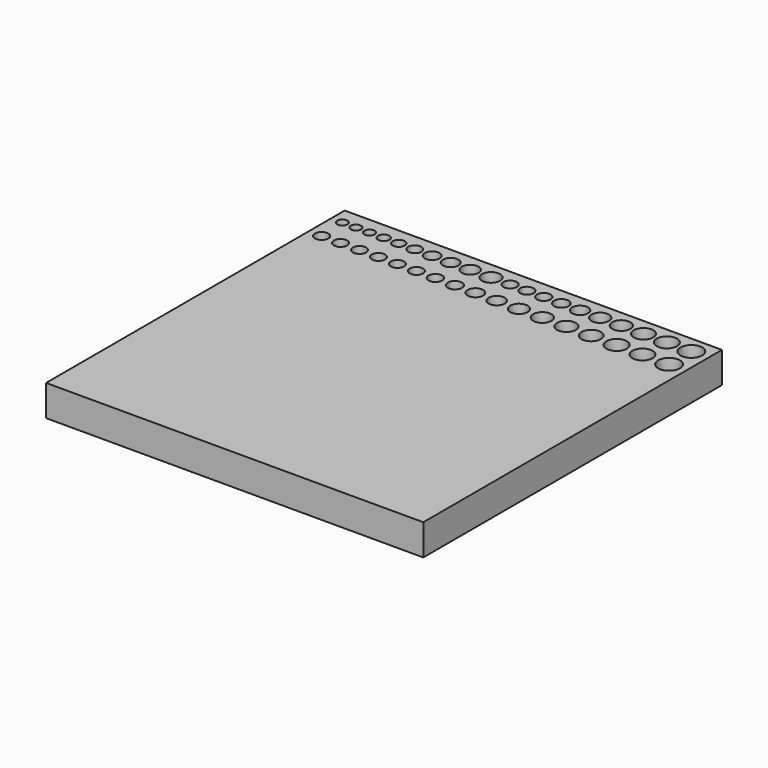
from build123d import *

# Parameters (mm, degrees)
F0_W     = 617.5375
F0_H     = 611.12411
F1_DEPTH = 50.8
F2_DEPTH = 25.4


# Not quite as in the source:
# - the dataset's text gives a spline's control points without its knots; the knots are read off the source's solid


with BuildPart() as f1:
    # F0 (on Top) → F1 (new body)
    with BuildSketch(Plane.XY):
        Rectangle(F0_W, F0_H)
        with BuildLine():
            add(Edge.make_bspline(
                [(-298.769016, 232.10194), (-298.769016, 238.169097), (-293.850797, 243.087316), (-287.783984, 243.087316), (-281.716482, 243.087316), (-276.798953, 238.169097), (-276.798953, 232.10194), (-276.798953, 226.035126), (-281.716482, 221.117253), (-287.783984, 221.117253), (-293.850797, 221.117253), (-298.769016, 226.035126), (-298.769016, 232.10194)],
                knots=[0, 0, 0, 0, 1, 1, 1, 2, 2, 2, 3, 3, 3, 4, 4, 4, 4], degree=3))
        make_face(mode=Mode.SUBTRACT)
        with BuildLine():
            add(Edge.make_bspline(
                [(-267.73973, 232.10194), (-267.73973, 238.158073), (-262.831158, 243.067334), (-256.77468, 243.067334), (-250.718891, 243.067334), (-245.80963, 238.158073), (-245.80963, 232.10194), (-245.80963, 226.046151), (-250.718891, 221.137234), (-256.77468, 221.137234), (-262.831158, 221.137234), (-267.73973, 226.046151), (-267.73973, 232.10194)],
                knots=[0, 0, 0, 0, 1, 1, 1, 2, 2, 2, 3, 3, 3, 4, 4, 4, 4], degree=3))
        make_face(mode=Mode.SUBTRACT)
        with BuildLine():
            add(Edge.make_bspline(
                [(-298.769016, 277.737052), (-298.769016, 282.365194), (-295.017651, 286.117247), (-290.389165, 286.117247), (-285.761024, 286.117247), (-282.008971, 282.365194), (-282.008971, 277.737052), (-282.008971, 273.108911), (-285.761024, 269.356858), (-290.389165, 269.356858), (-295.017651, 269.356858), (-298.769016, 273.108911), (-298.769016, 277.737052)],
                knots=[0, 0, 0, 0, 1, 1, 1, 2, 2, 2, 3, 3, 3, 4, 4, 4, 4], degree=3))
        make_face(mode=Mode.SUBTRACT)
        with BuildLine():
            add(Edge.make_bspline(
                [(-276.498885, 277.737052), (-276.498885, 282.362438), (-272.749588, 286.11208), (-268.123858, 286.11208), (-263.498473, 286.11208), (-259.748831, 282.362438), (-259.748831, 277.737052), (-259.748831, 273.111667), (-263.498473, 269.362025), (-268.123858, 269.362025), (-272.749588, 269.362025), (-276.498885, 273.111667), (-276.498885, 277.737052)],
                knots=[0, 0, 0, 0, 1, 1, 1, 2, 2, 2, 3, 3, 3, 4, 4, 4, 4], degree=3))
        make_face(mode=Mode.SUBTRACT)
        with BuildLine():
            add(Edge.make_bspline(
                [(-254.238745, 277.737052), (-254.238745, 282.398611), (-250.460509, 286.177192), (-245.79895, 286.177192), (-241.137736, 286.177192), (-237.359155, 282.398611), (-237.359155, 277.737052), (-237.359155, 273.075838), (-241.137736, 269.296913), (-245.79895, 269.296913), (-250.460509, 269.296913), (-254.238745, 273.075838), (-254.238745, 277.737052)],
                knots=[0, 0, 0, 0, 1, 1, 1, 2, 2, 2, 3, 3, 3, 4, 4, 4, 4], degree=3))
        make_face(mode=Mode.SUBTRACT)
        with BuildLine():
            add(Edge.make_bspline(
                [(-236.750407, 232.10194), (-236.750407, 238.163585), (-231.837012, 243.077325), (-225.775711, 243.077325), (-219.71441, 243.077325), (-214.800325, 238.163585), (-214.800325, 232.10194), (-214.800325, 226.040639), (-219.71441, 221.127243), (-225.775711, 221.127243), (-231.837012, 221.127243), (-236.750407, 226.040639), (-236.750407, 232.10194)],
                knots=[0, 0, 0, 0, 1, 1, 1, 2, 2, 2, 3, 3, 3, 4, 4, 4, 4], degree=3))
        make_face(mode=Mode.SUBTRACT)
        with BuildLine():
            add(Edge.make_bspline(
                [(-205.741102, 232.102284), (-205.741102, 238.17771), (-200.816683, 243.102474), (-194.740912, 243.102474), (-188.665831, 243.102474), (-183.741412, 238.17771), (-183.741412, 232.102284), (-183.741412, 226.027203), (-188.665831, 221.102439), (-194.740912, 221.102439), (-200.816683, 221.102439), (-205.741102, 226.027203), (-205.741102, 232.102284)],
                knots=[0, 0, 0, 0, 1, 1, 1, 2, 2, 2, 3, 3, 3, 4, 4, 4, 4], degree=3))
        make_face(mode=Mode.SUBTRACT)
        with BuildLine():
            add(Edge.make_bspline(
                [(-174.682188, 232.10194), (-174.682188, 238.17771), (-169.75708, 243.102474), (-163.681999, 243.102474), (-157.606917, 243.102474), (-152.681809, 238.17771), (-152.681809, 232.10194), (-152.681809, 226.026858), (-157.606917, 221.102094), (-163.681999, 221.102094), (-169.75708, 221.102094), (-174.682188, 226.026858), (-174.682188, 232.10194)],
                knots=[0, 0, 0, 0, 1, 1, 1, 2, 2, 2, 3, 3, 3, 4, 4, 4, 4], degree=3))
        make_face(mode=Mode.SUBTRACT)
        with BuildLine():
            add(Edge.make_bspline(
                [(-231.849414, 277.73688), (-231.849414, 282.848368), (-227.705998, 286.992129), (-222.594509, 286.992129), (-217.482677, 286.992129), (-213.33926, 282.848368), (-213.33926, 277.73688), (-213.33926, 272.625392), (-217.482677, 268.481976), (-222.594509, 268.481976), (-227.705998, 268.481976), (-231.849414, 272.625392), (-231.849414, 277.73688)],
                knots=[0, 0, 0, 0, 1, 1, 1, 2, 2, 2, 3, 3, 3, 4, 4, 4, 4], degree=3))
        make_face(mode=Mode.SUBTRACT)
        with BuildLine():
            add(Edge.make_bspline(
                [(-198.029256179, 287.5369713483), (-192.616666179, 287.5369712893), (-188.2293372268, 283.1496422416), (-188.2293372857, 277.7370522416), (-188.2293373447, 272.3244632416), (-192.6166663924, 267.9371332893), (-198.0292563924, 267.9371333483), (-203.4418453924, 267.9371334072), (-207.8291743447, 272.324463455), (-207.8291742857, 277.737052455), (-207.8291742268, 283.149642455), (-203.441845179, 287.5369714072), (-198.029256179, 287.5369713483)],
                knots=[0, 0, 0, 0, 1, 1, 1, 2, 2, 2, 3, 3, 3, 4, 4, 4, 4], degree=3))
        make_face(mode=Mode.SUBTRACT)
        with BuildLine():
            add(Edge.make_bspline(
                [(-182.719596, 277.737052), (-182.719596, 283.759424), (-177.837207, 288.641813), (-171.814491, 288.641813), (-165.792464, 288.641813), (-160.90973, 283.759424), (-160.90973, 277.737052), (-160.90973, 271.714681), (-165.792464, 266.832292), (-171.814491, 266.832292), (-177.837207, 266.832292), (-182.719596, 271.714681), (-182.719596, 277.737052)],
                knots=[0, 0, 0, 0, 1, 1, 1, 2, 2, 2, 3, 3, 3, 4, 4, 4, 4], degree=3))
        make_face(mode=Mode.SUBTRACT)
        with BuildLine():
            add(Edge.make_bspline(
                [(-143.622586, 232.10194), (-143.622586, 238.144293), (-138.725038, 243.042529), (-132.68234, 243.042529), (-126.640332, 243.042529), (-121.742784, 238.144293), (-121.742784, 232.10194), (-121.742784, 226.059931), (-126.640332, 221.162039), (-132.68234, 221.162039), (-138.725038, 221.162039), (-143.622586, 226.059931), (-143.622586, 232.10194)],
                knots=[0, 0, 0, 0, 1, 1, 1, 2, 2, 2, 3, 3, 3, 4, 4, 4, 4], degree=3))
        make_face(mode=Mode.SUBTRACT)
        with BuildLine():
            add(Edge.make_bspline(
                [(-112.683561, 232.102284), (-112.683561, 238.260737), (-107.692307, 243.25268), (-101.533854, 243.25268), (-95.375401, 243.25268), (-90.383458, 238.260737), (-90.383458, 232.102284), (-90.383458, 225.94452), (-95.375401, 220.952233), (-101.533854, 220.952233), (-107.692307, 220.952233), (-112.683561, 225.94452), (-112.683561, 232.102284)],
                knots=[0, 0, 0, 0, 1, 1, 1, 2, 2, 2, 3, 3, 3, 4, 4, 4, 4], degree=3))
        make_face(mode=Mode.SUBTRACT)
        with BuildLine():
            add(Edge.make_bspline(
                [(-155.399645, 277.737052), (-155.399645, 284.402968), (-149.995668, 289.806945), (-143.329408, 289.806945), (-136.663837, 289.806945), (-131.259516, 284.402968), (-131.259516, 277.737052), (-131.259516, 271.071137), (-136.663837, 265.66716), (-143.329408, 265.66716), (-149.995668, 265.66716), (-155.399645, 271.071137), (-155.399645, 277.737052)],
                knots=[0, 0, 0, 0, 1, 1, 1, 2, 2, 2, 3, 3, 3, 4, 4, 4, 4], degree=3))
        make_face(mode=Mode.SUBTRACT)
        with BuildLine():
            add(Edge.make_bspline(
                [(-112.9898302501, 290.4969974494), (-105.9425422501, 290.4969974298), (-100.2298852661, 284.7843394139), (-100.2298852857, 277.7370524139), (-100.2298853054, 270.6897654139), (-105.9425423213, 264.9771074298), (-112.9898303213, 264.9771074494), (-120.0371173213, 264.9771074691), (-125.7497743054, 270.689765485), (-125.7497742857, 277.737052485), (-125.7497742661, 284.784339485), (-120.0371172501, 290.4969974691), (-112.9898302501, 290.4969974494)],
                knots=[0, 0, 0, 0, 1, 1, 1, 2, 2, 2, 3, 3, 3, 4, 4, 4, 4], degree=3))
        make_face(mode=Mode.SUBTRACT)
        with BuildLine():
            add(Edge.make_bspline(
                [(-94.7198, 277.737052), (-94.7198, 285.305927), (-88.584085, 291.441987), (-81.014865, 291.441987), (-73.446335, 291.441987), (-67.309931, 285.305927), (-67.309931, 277.737052), (-67.309931, 270.168178), (-73.446335, 264.032118), (-81.014865, 264.032118), (-88.584085, 264.032118), (-94.7198, 270.168178), (-94.7198, 277.737052)],
                knots=[0, 0, 0, 0, 1, 1, 1, 2, 2, 2, 3, 3, 3, 4, 4, 4, 4], degree=3))
        make_face(mode=Mode.SUBTRACT)
        with BuildLine():
            add(Edge.make_bspline(
                [(-81.324235, 232.102284), (-81.324235, 238.583887), (-76.071153, 243.837657), (-69.589551, 243.837657), (-63.107948, 243.837657), (-57.854177, 238.583887), (-57.854177, 232.102284), (-57.854177, 225.621371), (-63.107948, 220.367255), (-69.589551, 220.367255), (-76.071153, 220.367255), (-81.324235, 225.621371), (-81.324235, 232.102284)],
                knots=[0, 0, 0, 0, 1, 1, 1, 2, 2, 2, 3, 3, 3, 4, 4, 4, 4], degree=3))
        make_face(mode=Mode.SUBTRACT)
        with BuildLine():
            add(Edge.make_bspline(
                [(-48.794954, 232.10194), (-48.794954, 239.11891), (-43.106413, 244.807107), (-36.089442, 244.807107), (-29.073161, 244.807107), (-23.384619, 239.11891), (-23.384619, 232.10194), (-23.384619, 225.085658), (-29.073161, 219.397461), (-36.089442, 219.397461), (-43.106413, 219.397461), (-48.794954, 225.085658), (-48.794954, 232.10194)],
                knots=[0, 0, 0, 0, 1, 1, 1, 2, 2, 2, 3, 3, 3, 4, 4, 4, 4], degree=3))
        make_face(mode=Mode.SUBTRACT)
        with BuildLine():
            add(Edge.make_bspline(
                [(-14.325396, 232.10194), (-14.325396, 239.353866), (-8.447374, 245.232232), (-1.195448, 245.232232), (6.055789, 245.232232), (11.9345, 239.353866), (11.9345, 232.10194), (11.9345, 224.850703), (6.055789, 218.971992), (-1.195448, 218.971992), (-8.447374, 218.971992), (-14.325396, 224.850703), (-14.325396, 232.10194)],
                knots=[0, 0, 0, 0, 1, 1, 1, 2, 2, 2, 3, 3, 3, 4, 4, 4, 4], degree=3))
        make_face(mode=Mode.SUBTRACT)
        with BuildLine():
            add(Edge.make_bspline(
                [(-61.80019, 277.737052), (-61.80019, 285.919154), (-55.167347, 292.551997), (-46.985246, 292.551997), (-38.803144, 292.551997), (-32.169957, 285.919154), (-32.169957, 277.737052), (-32.169957, 269.554951), (-38.803144, 262.922108), (-46.985246, 262.922108), (-55.167347, 262.922108), (-61.80019, 269.554951), (-61.80019, 277.737052)],
                knots=[0, 0, 0, 0, 1, 1, 1, 2, 2, 2, 3, 3, 3, 4, 4, 4, 4], degree=3))
        make_face(mode=Mode.SUBTRACT)
        with BuildLine():
            add(Edge.make_bspline(
                [(-26.66056, 277.737052), (-26.66056, 283.80111), (-21.745098, 288.716916), (-15.681041, 288.716916), (-9.616984, 288.716916), (-4.700833, 283.80111), (-4.700833, 277.737052), (-4.700833, 271.672995), (-9.616984, 266.757189), (-15.681041, 266.757189), (-21.745098, 266.757189), (-26.66056, 271.672995), (-26.66056, 277.737052)],
                knots=[0, 0, 0, 0, 1, 1, 1, 2, 2, 2, 3, 3, 3, 4, 4, 4, 4], degree=3))
        make_face(mode=Mode.SUBTRACT)
        with BuildLine():
            add(Edge.make_bspline(
                [(20.993723, 232.101595), (20.993723, 239.974672), (27.375762, 246.357056), (35.248495, 246.357056), (43.120882, 246.357056), (49.503266, 239.974672), (49.503266, 232.101595), (49.503266, 224.229207), (43.120882, 217.846824), (35.248495, 217.846824), (27.375762, 217.846824), (20.993723, 224.229207), (20.993723, 232.101595)],
                knots=[0, 0, 0, 0, 1, 1, 1, 2, 2, 2, 3, 3, 3, 4, 4, 4, 4], degree=3))
        make_face(mode=Mode.SUBTRACT)
        with BuildLine():
            add(Edge.make_bspline(
                [(58.562489, 232.101595), (58.562489, 240.350187), (65.249075, 247.037118), (73.497667, 247.037118), (81.74557, 247.037118), (88.432501, 240.350187), (88.432501, 232.101595), (88.432501, 223.853692), (81.74557, 217.166762), (73.497667, 217.166762), (65.249075, 217.166762), (58.562489, 223.853692), (58.562489, 232.101595)],
                knots=[0, 0, 0, 0, 1, 1, 1, 2, 2, 2, 3, 3, 3, 4, 4, 4, 4], degree=3))
        make_face(mode=Mode.SUBTRACT)
        with BuildLine():
            add(Edge.make_bspline(
                [(0.808908, 277.737052), (0.808908, 283.812134), (5.733328, 288.736898), (11.809098, 288.736898), (17.88418, 288.736898), (22.808599, 283.812134), (22.808599, 277.737052), (22.808599, 271.661971), (17.88418, 266.737207), (11.809098, 266.737207), (5.733328, 266.737207), (0.808908, 271.661971), (0.808908, 277.737052)],
                knots=[0, 0, 0, 0, 1, 1, 1, 2, 2, 2, 3, 3, 3, 4, 4, 4, 4], degree=3))
        make_face(mode=Mode.SUBTRACT)
        with BuildLine():
            add(Edge.make_bspline(
                [(28.318685, 277.737052), (28.318685, 283.87828), (33.296848, 288.857132), (39.438764, 288.857132), (45.579991, 288.857132), (50.558843, 283.87828), (50.558843, 277.737052), (50.558843, 271.595825), (45.579991, 266.616973), (39.438764, 266.616973), (33.296848, 266.616973), (28.318685, 271.595825), (28.318685, 277.737052)],
                knots=[0, 0, 0, 0, 1, 1, 1, 2, 2, 2, 3, 3, 3, 4, 4, 4, 4], degree=3))
        make_face(mode=Mode.SUBTRACT)
        with BuildLine():
            add(Edge.make_bspline(
                [(56.068929, 277.737052), (56.068929, 284.380919), (61.454991, 289.766981), (68.099203, 289.766981), (74.742725, 289.766981), (80.128787, 284.380919), (80.128787, 277.737052), (80.128787, 271.093186), (74.742725, 265.707124), (68.099203, 265.707124), (61.454991, 265.707124), (56.068929, 271.093186), (56.068929, 277.737052)],
                knots=[0, 0, 0, 0, 1, 1, 1, 2, 2, 2, 3, 3, 3, 4, 4, 4, 4], degree=3))
        make_face(mode=Mode.SUBTRACT)
        with BuildLine():
            add(Edge.make_bspline(
                [(97.491724, 232.10194), (97.491724, 240.673682), (104.440481, 247.622095), (113.011879, 247.622095), (121.583276, 247.622095), (128.532034, 240.673682), (128.532034, 232.10194), (128.532034, 223.530542), (121.583276, 216.582129), (113.011879, 216.582129), (104.440481, 216.582129), (97.491724, 223.530542), (97.491724, 232.10194)],
                knots=[0, 0, 0, 0, 1, 1, 1, 2, 2, 2, 3, 3, 3, 4, 4, 4, 4], degree=3))
        make_face(mode=Mode.SUBTRACT)
        with BuildLine():
            add(Edge.make_bspline(
                [(137.591257, 232.101595), (137.591257, 240.883488), (144.710202, 248.002089), (153.491062, 248.002089), (162.27261, 248.002089), (169.390866, 240.883488), (169.390866, 232.101595), (169.390866, 223.320736), (162.27261, 216.20179), (153.491062, 216.20179), (144.710202, 216.20179), (137.591257, 223.320736), (137.591257, 232.101595)],
                knots=[0, 0, 0, 0, 1, 1, 1, 2, 2, 2, 3, 3, 3, 4, 4, 4, 4], degree=3))
        make_face(mode=Mode.SUBTRACT)
        with BuildLine():
            add(Edge.make_bspline(
                [(85.638873, 277.737052), (85.638873, 284.994146), (91.521718, 290.876991), (98.778467, 290.876991), (106.035216, 290.876991), (111.91875, 284.994146), (111.91875, 277.737052), (111.91875, 270.479959), (106.035216, 264.597114), (98.778467, 264.597114), (91.521718, 264.597114), (85.638873, 270.479959), (85.638873, 277.737052)],
                knots=[0, 0, 0, 0, 1, 1, 1, 2, 2, 2, 3, 3, 3, 4, 4, 4, 4], degree=3))
        make_face(mode=Mode.SUBTRACT)
        with BuildLine():
            add(Edge.make_bspline(
                [(117.428836, 277.737052), (117.428836, 285.615297), (123.815354, 292.002159), (131.694287, 292.002159), (139.572531, 292.002159), (145.959049, 285.615297), (145.959049, 277.737052), (145.959049, 269.858808), (139.572531, 263.471946), (131.694287, 263.471946), (123.815354, 263.471946), (117.428836, 269.858808), (117.428836, 277.737052)],
                knots=[0, 0, 0, 0, 1, 1, 1, 2, 2, 2, 3, 3, 3, 4, 4, 4, 4], degree=3))
        make_face(mode=Mode.SUBTRACT)
        with BuildLine():
            add(Edge.make_bspline(
                [(178.45009, 232.10194), (178.45009, 241.336518), (185.935593, 248.822022), (195.170516, 248.822022), (204.40475, 248.822022), (211.890253, 241.336518), (211.890253, 232.10194), (211.890253, 222.86805), (204.40475, 215.382202), (195.170516, 215.382202), (185.935593, 215.382202), (178.45009, 222.86805), (178.45009, 232.10194)],
                knots=[0, 0, 0, 0, 1, 1, 1, 2, 2, 2, 3, 3, 3, 4, 4, 4, 4], degree=3))
        make_face(mode=Mode.SUBTRACT)
        with BuildLine():
            add(Edge.make_bspline(
                [(151.468791, 277.737052), (151.468791, 285.935691), (158.115069, 292.581969), (166.314052, 292.581969), (174.512345, 292.581969), (181.158624, 285.935691), (181.158624, 277.737052), (181.158624, 269.538414), (174.512345, 262.892136), (166.314052, 262.892136), (158.115069, 262.892136), (151.468791, 269.538414), (151.468791, 277.737052)],
                knots=[0, 0, 0, 0, 1, 1, 1, 2, 2, 2, 3, 3, 3, 4, 4, 4, 4], degree=3))
        make_face(mode=Mode.SUBTRACT)
        with BuildLine():
            add(Edge.make_bspline(
                [(202.6784122857, 293.7471), (211.5205952857, 293.7471), (218.6884602857, 286.579235), (218.6884602857, 277.737052), (218.6884602857, 268.89487), (211.5205952857, 261.727005), (202.6784122857, 261.727005), (193.8362302857, 261.727005), (186.6683652857, 268.89487), (186.6683652857, 277.737052), (186.6683652857, 286.579235), (193.8362302857, 293.7471), (202.6784122857, 293.7471)],
                knots=[0, 0, 0, 0, 1, 1, 1, 2, 2, 2, 3, 3, 3, 4, 4, 4, 4], degree=3))
        make_face(mode=Mode.SUBTRACT)
        with BuildLine():
            add(Edge.make_bspline(
                [(220.949476, 232.10194), (220.949476, 241.253491), (228.368145, 248.67216), (237.519697, 248.67216), (246.670904, 248.67216), (254.089572, 241.253491), (254.089572, 232.10194), (254.089572, 222.951077), (246.670904, 215.532064), (237.519697, 215.532064), (228.368145, 215.532064), (220.949476, 222.951077), (220.949476, 232.10194)],
                knots=[0, 0, 0, 0, 1, 1, 1, 2, 2, 2, 3, 3, 3, 4, 4, 4, 4], degree=3))
        make_face(mode=Mode.SUBTRACT)
        with BuildLine():
            add(Edge.make_bspline(
                [(263.148796, 232.101595), (263.148796, 241.938032), (271.122814, 249.91205), (280.95925, 249.91205), (290.794998, 249.91205), (298.769016, 241.938032), (298.769016, 232.101595), (298.769016, 222.265503), (290.794998, 214.29183), (280.95925, 214.29183), (271.122814, 214.29183), (263.148796, 222.265503), (263.148796, 232.101595)],
                knots=[0, 0, 0, 0, 1, 1, 1, 2, 2, 2, 3, 3, 3, 4, 4, 4, 4], degree=3))
        make_face(mode=Mode.SUBTRACT)
        with BuildLine():
            add(Edge.make_bspline(
                [(224.198546, 277.737052), (224.198546, 286.963018), (231.677848, 294.441976), (240.903814, 294.441976), (250.12978, 294.441976), (257.608393, 286.963018), (257.608393, 277.737052), (257.608393, 268.511087), (250.12978, 261.032129), (240.903814, 261.032129), (231.677848, 261.032129), (224.198546, 268.511087), (224.198546, 277.737052)],
                knots=[0, 0, 0, 0, 1, 1, 1, 2, 2, 2, 3, 3, 3, 4, 4, 4, 4], degree=3))
        make_face(mode=Mode.SUBTRACT)
        with BuildLine():
            add(Edge.make_bspline(
                [(263.118479, 277.737052), (263.118479, 287.581413), (271.098698, 295.561977), (280.943403, 295.561977), (290.788108, 295.561977), (298.768327, 287.581413), (298.768327, 277.737052), (298.768327, 267.892692), (290.788108, 259.912128), (280.943403, 259.912128), (271.098698, 259.912128), (263.118479, 267.892692), (263.118479, 277.737052)],
                knots=[0, 0, 0, 0, 1, 1, 1, 2, 2, 2, 3, 3, 3, 4, 4, 4, 4], degree=3))
        make_face(mode=Mode.SUBTRACT)
        with BuildLine():
            add(Edge.make_bspline(
                [(263.118479, 277.737052), (263.118479, 287.581413), (271.098698, 295.561977), (280.943403, 295.561977), (290.788108, 295.561977), (298.768327, 287.581413), (298.768327, 277.737052), (298.768327, 267.892692), (290.788108, 259.912128), (280.943403, 259.912128), (271.098698, 259.912128), (263.118479, 267.892692), (263.118479, 277.737052)],
                knots=[0, 0, 0, 0, 1, 1, 1, 2, 2, 2, 3, 3, 3, 4, 4, 4, 4], degree=3))
        make_face()
        with BuildLine():
            add(Edge.make_bspline(
                [(263.148796, 232.101595), (263.148796, 241.938032), (271.122814, 249.91205), (280.95925, 249.91205), (290.794998, 249.91205), (298.769016, 241.938032), (298.769016, 232.101595), (298.769016, 222.265503), (290.794998, 214.29183), (280.95925, 214.29183), (271.122814, 214.29183), (263.148796, 222.265503), (263.148796, 232.101595)],
                knots=[0, 0, 0, 0, 1, 1, 1, 2, 2, 2, 3, 3, 3, 4, 4, 4, 4], degree=3))
        make_face()
        with BuildLine():
            add(Edge.make_bspline(
                [(178.45009, 232.10194), (178.45009, 241.336518), (185.935593, 248.822022), (195.170516, 248.822022), (204.40475, 248.822022), (211.890253, 241.336518), (211.890253, 232.10194), (211.890253, 222.86805), (204.40475, 215.382202), (195.170516, 215.382202), (185.935593, 215.382202), (178.45009, 222.86805), (178.45009, 232.10194)],
                knots=[0, 0, 0, 0, 1, 1, 1, 2, 2, 2, 3, 3, 3, 4, 4, 4, 4], degree=3))
        make_face()
        with BuildLine():
            add(Edge.make_bspline(
                [(224.198546, 277.737052), (224.198546, 286.963018), (231.677848, 294.441976), (240.903814, 294.441976), (250.12978, 294.441976), (257.608393, 286.963018), (257.608393, 277.737052), (257.608393, 268.511087), (250.12978, 261.032129), (240.903814, 261.032129), (231.677848, 261.032129), (224.198546, 268.511087), (224.198546, 277.737052)],
                knots=[0, 0, 0, 0, 1, 1, 1, 2, 2, 2, 3, 3, 3, 4, 4, 4, 4], degree=3))
        make_face()
        with BuildLine():
            add(Edge.make_bspline(
                [(220.949476, 232.10194), (220.949476, 241.253491), (228.368145, 248.67216), (237.519697, 248.67216), (246.670904, 248.67216), (254.089572, 241.253491), (254.089572, 232.10194), (254.089572, 222.951077), (246.670904, 215.532064), (237.519697, 215.532064), (228.368145, 215.532064), (220.949476, 222.951077), (220.949476, 232.10194)],
                knots=[0, 0, 0, 0, 1, 1, 1, 2, 2, 2, 3, 3, 3, 4, 4, 4, 4], degree=3))
        make_face()
        with BuildLine():
            add(Edge.make_bspline(
                [(202.6784122857, 293.7471), (211.5205952857, 293.7471), (218.6884602857, 286.579235), (218.6884602857, 277.737052), (218.6884602857, 268.89487), (211.5205952857, 261.727005), (202.6784122857, 261.727005), (193.8362302857, 261.727005), (186.6683652857, 268.89487), (186.6683652857, 277.737052), (186.6683652857, 286.579235), (193.8362302857, 293.7471), (202.6784122857, 293.7471)],
                knots=[0, 0, 0, 0, 1, 1, 1, 2, 2, 2, 3, 3, 3, 4, 4, 4, 4], degree=3))
        make_face()
        with BuildLine():
            add(Edge.make_bspline(
                [(137.591257, 232.101595), (137.591257, 240.883488), (144.710202, 248.002089), (153.491062, 248.002089), (162.27261, 248.002089), (169.390866, 240.883488), (169.390866, 232.101595), (169.390866, 223.320736), (162.27261, 216.20179), (153.491062, 216.20179), (144.710202, 216.20179), (137.591257, 223.320736), (137.591257, 232.101595)],
                knots=[0, 0, 0, 0, 1, 1, 1, 2, 2, 2, 3, 3, 3, 4, 4, 4, 4], degree=3))
        make_face()
        with BuildLine():
            add(Edge.make_bspline(
                [(97.491724, 232.10194), (97.491724, 240.673682), (104.440481, 247.622095), (113.011879, 247.622095), (121.583276, 247.622095), (128.532034, 240.673682), (128.532034, 232.10194), (128.532034, 223.530542), (121.583276, 216.582129), (113.011879, 216.582129), (104.440481, 216.582129), (97.491724, 223.530542), (97.491724, 232.10194)],
                knots=[0, 0, 0, 0, 1, 1, 1, 2, 2, 2, 3, 3, 3, 4, 4, 4, 4], degree=3))
        make_face()
        with BuildLine():
            add(Edge.make_bspline(
                [(58.562489, 232.101595), (58.562489, 240.350187), (65.249075, 247.037118), (73.497667, 247.037118), (81.74557, 247.037118), (88.432501, 240.350187), (88.432501, 232.101595), (88.432501, 223.853692), (81.74557, 217.166762), (73.497667, 217.166762), (65.249075, 217.166762), (58.562489, 223.853692), (58.562489, 232.101595)],
                knots=[0, 0, 0, 0, 1, 1, 1, 2, 2, 2, 3, 3, 3, 4, 4, 4, 4], degree=3))
        make_face()
        with BuildLine():
            add(Edge.make_bspline(
                [(151.468791, 277.737052), (151.468791, 285.935691), (158.115069, 292.581969), (166.314052, 292.581969), (174.512345, 292.581969), (181.158624, 285.935691), (181.158624, 277.737052), (181.158624, 269.538414), (174.512345, 262.892136), (166.314052, 262.892136), (158.115069, 262.892136), (151.468791, 269.538414), (151.468791, 277.737052)],
                knots=[0, 0, 0, 0, 1, 1, 1, 2, 2, 2, 3, 3, 3, 4, 4, 4, 4], degree=3))
        make_face()
        with BuildLine():
            add(Edge.make_bspline(
                [(-61.80019, 277.737052), (-61.80019, 285.919154), (-55.167347, 292.551997), (-46.985246, 292.551997), (-38.803144, 292.551997), (-32.169957, 285.919154), (-32.169957, 277.737052), (-32.169957, 269.554951), (-38.803144, 262.922108), (-46.985246, 262.922108), (-55.167347, 262.922108), (-61.80019, 269.554951), (-61.80019, 277.737052)],
                knots=[0, 0, 0, 0, 1, 1, 1, 2, 2, 2, 3, 3, 3, 4, 4, 4, 4], degree=3))
        make_face()
        with BuildLine():
            add(Edge.make_bspline(
                [(117.428836, 277.737052), (117.428836, 285.615297), (123.815354, 292.002159), (131.694287, 292.002159), (139.572531, 292.002159), (145.959049, 285.615297), (145.959049, 277.737052), (145.959049, 269.858808), (139.572531, 263.471946), (131.694287, 263.471946), (123.815354, 263.471946), (117.428836, 269.858808), (117.428836, 277.737052)],
                knots=[0, 0, 0, 0, 1, 1, 1, 2, 2, 2, 3, 3, 3, 4, 4, 4, 4], degree=3))
        make_face()
        with BuildLine():
            add(Edge.make_bspline(
                [(20.993723, 232.101595), (20.993723, 239.974672), (27.375762, 246.357056), (35.248495, 246.357056), (43.120882, 246.357056), (49.503266, 239.974672), (49.503266, 232.101595), (49.503266, 224.229207), (43.120882, 217.846824), (35.248495, 217.846824), (27.375762, 217.846824), (20.993723, 224.229207), (20.993723, 232.101595)],
                knots=[0, 0, 0, 0, 1, 1, 1, 2, 2, 2, 3, 3, 3, 4, 4, 4, 4], degree=3))
        make_face()
        with BuildLine():
            add(Edge.make_bspline(
                [(-94.7198, 277.737052), (-94.7198, 285.305927), (-88.584085, 291.441987), (-81.014865, 291.441987), (-73.446335, 291.441987), (-67.309931, 285.305927), (-67.309931, 277.737052), (-67.309931, 270.168178), (-73.446335, 264.032118), (-81.014865, 264.032118), (-88.584085, 264.032118), (-94.7198, 270.168178), (-94.7198, 277.737052)],
                knots=[0, 0, 0, 0, 1, 1, 1, 2, 2, 2, 3, 3, 3, 4, 4, 4, 4], degree=3))
        make_face()
        with BuildLine():
            add(Edge.make_bspline(
                [(85.638873, 277.737052), (85.638873, 284.994146), (91.521718, 290.876991), (98.778467, 290.876991), (106.035216, 290.876991), (111.91875, 284.994146), (111.91875, 277.737052), (111.91875, 270.479959), (106.035216, 264.597114), (98.778467, 264.597114), (91.521718, 264.597114), (85.638873, 270.479959), (85.638873, 277.737052)],
                knots=[0, 0, 0, 0, 1, 1, 1, 2, 2, 2, 3, 3, 3, 4, 4, 4, 4], degree=3))
        make_face()
        with BuildLine():
            add(Edge.make_bspline(
                [(-14.325396, 232.10194), (-14.325396, 239.353866), (-8.447374, 245.232232), (-1.195448, 245.232232), (6.055789, 245.232232), (11.9345, 239.353866), (11.9345, 232.10194), (11.9345, 224.850703), (6.055789, 218.971992), (-1.195448, 218.971992), (-8.447374, 218.971992), (-14.325396, 224.850703), (-14.325396, 232.10194)],
                knots=[0, 0, 0, 0, 1, 1, 1, 2, 2, 2, 3, 3, 3, 4, 4, 4, 4], degree=3))
        make_face()
        with BuildLine():
            add(Edge.make_bspline(
                [(-112.9898302501, 290.4969974494), (-105.9425422501, 290.4969974298), (-100.2298852661, 284.7843394139), (-100.2298852857, 277.7370524139), (-100.2298853054, 270.6897654139), (-105.9425423213, 264.9771074298), (-112.9898303213, 264.9771074494), (-120.0371173213, 264.9771074691), (-125.7497743054, 270.689765485), (-125.7497742857, 277.737052485), (-125.7497742661, 284.784339485), (-120.0371172501, 290.4969974691), (-112.9898302501, 290.4969974494)],
                knots=[0, 0, 0, 0, 1, 1, 1, 2, 2, 2, 3, 3, 3, 4, 4, 4, 4], degree=3))
        make_face()
        with BuildLine():
            add(Edge.make_bspline(
                [(-48.794954, 232.10194), (-48.794954, 239.11891), (-43.106413, 244.807107), (-36.089442, 244.807107), (-29.073161, 244.807107), (-23.384619, 239.11891), (-23.384619, 232.10194), (-23.384619, 225.085658), (-29.073161, 219.397461), (-36.089442, 219.397461), (-43.106413, 219.397461), (-48.794954, 225.085658), (-48.794954, 232.10194)],
                knots=[0, 0, 0, 0, 1, 1, 1, 2, 2, 2, 3, 3, 3, 4, 4, 4, 4], degree=3))
        make_face()
        with BuildLine():
            add(Edge.make_bspline(
                [(-155.399645, 277.737052), (-155.399645, 284.402968), (-149.995668, 289.806945), (-143.329408, 289.806945), (-136.663837, 289.806945), (-131.259516, 284.402968), (-131.259516, 277.737052), (-131.259516, 271.071137), (-136.663837, 265.66716), (-143.329408, 265.66716), (-149.995668, 265.66716), (-155.399645, 271.071137), (-155.399645, 277.737052)],
                knots=[0, 0, 0, 0, 1, 1, 1, 2, 2, 2, 3, 3, 3, 4, 4, 4, 4], degree=3))
        make_face()
        with BuildLine():
            add(Edge.make_bspline(
                [(56.068929, 277.737052), (56.068929, 284.380919), (61.454991, 289.766981), (68.099203, 289.766981), (74.742725, 289.766981), (80.128787, 284.380919), (80.128787, 277.737052), (80.128787, 271.093186), (74.742725, 265.707124), (68.099203, 265.707124), (61.454991, 265.707124), (56.068929, 271.093186), (56.068929, 277.737052)],
                knots=[0, 0, 0, 0, 1, 1, 1, 2, 2, 2, 3, 3, 3, 4, 4, 4, 4], degree=3))
        make_face()
        with BuildLine():
            add(Edge.make_bspline(
                [(-81.324235, 232.102284), (-81.324235, 238.583887), (-76.071153, 243.837657), (-69.589551, 243.837657), (-63.107948, 243.837657), (-57.854177, 238.583887), (-57.854177, 232.102284), (-57.854177, 225.621371), (-63.107948, 220.367255), (-69.589551, 220.367255), (-76.071153, 220.367255), (-81.324235, 225.621371), (-81.324235, 232.102284)],
                knots=[0, 0, 0, 0, 1, 1, 1, 2, 2, 2, 3, 3, 3, 4, 4, 4, 4], degree=3))
        make_face()
        with BuildLine():
            add(Edge.make_bspline(
                [(-112.683561, 232.102284), (-112.683561, 238.260737), (-107.692307, 243.25268), (-101.533854, 243.25268), (-95.375401, 243.25268), (-90.383458, 238.260737), (-90.383458, 232.102284), (-90.383458, 225.94452), (-95.375401, 220.952233), (-101.533854, 220.952233), (-107.692307, 220.952233), (-112.683561, 225.94452), (-112.683561, 232.102284)],
                knots=[0, 0, 0, 0, 1, 1, 1, 2, 2, 2, 3, 3, 3, 4, 4, 4, 4], degree=3))
        make_face()
        with BuildLine():
            add(Edge.make_bspline(
                [(28.318685, 277.737052), (28.318685, 283.87828), (33.296848, 288.857132), (39.438764, 288.857132), (45.579991, 288.857132), (50.558843, 283.87828), (50.558843, 277.737052), (50.558843, 271.595825), (45.579991, 266.616973), (39.438764, 266.616973), (33.296848, 266.616973), (28.318685, 271.595825), (28.318685, 277.737052)],
                knots=[0, 0, 0, 0, 1, 1, 1, 2, 2, 2, 3, 3, 3, 4, 4, 4, 4], degree=3))
        make_face()
        with BuildLine():
            add(Edge.make_bspline(
                [(-174.682188, 232.10194), (-174.682188, 238.17771), (-169.75708, 243.102474), (-163.681999, 243.102474), (-157.606917, 243.102474), (-152.681809, 238.17771), (-152.681809, 232.10194), (-152.681809, 226.026858), (-157.606917, 221.102094), (-163.681999, 221.102094), (-169.75708, 221.102094), (-174.682188, 226.026858), (-174.682188, 232.10194)],
                knots=[0, 0, 0, 0, 1, 1, 1, 2, 2, 2, 3, 3, 3, 4, 4, 4, 4], degree=3))
        make_face()
        with BuildLine():
            add(Edge.make_bspline(
                [(-205.741102, 232.102284), (-205.741102, 238.17771), (-200.816683, 243.102474), (-194.740912, 243.102474), (-188.665831, 243.102474), (-183.741412, 238.17771), (-183.741412, 232.102284), (-183.741412, 226.027203), (-188.665831, 221.102439), (-194.740912, 221.102439), (-200.816683, 221.102439), (-205.741102, 226.027203), (-205.741102, 232.102284)],
                knots=[0, 0, 0, 0, 1, 1, 1, 2, 2, 2, 3, 3, 3, 4, 4, 4, 4], degree=3))
        make_face()
        with BuildLine():
            add(Edge.make_bspline(
                [(0.808908, 277.737052), (0.808908, 283.812134), (5.733328, 288.736898), (11.809098, 288.736898), (17.88418, 288.736898), (22.808599, 283.812134), (22.808599, 277.737052), (22.808599, 271.661971), (17.88418, 266.737207), (11.809098, 266.737207), (5.733328, 266.737207), (0.808908, 271.661971), (0.808908, 277.737052)],
                knots=[0, 0, 0, 0, 1, 1, 1, 2, 2, 2, 3, 3, 3, 4, 4, 4, 4], degree=3))
        make_face()
        with BuildLine():
            add(Edge.make_bspline(
                [(-298.769016, 232.10194), (-298.769016, 238.169097), (-293.850797, 243.087316), (-287.783984, 243.087316), (-281.716482, 243.087316), (-276.798953, 238.169097), (-276.798953, 232.10194), (-276.798953, 226.035126), (-281.716482, 221.117253), (-287.783984, 221.117253), (-293.850797, 221.117253), (-298.769016, 226.035126), (-298.769016, 232.10194)],
                knots=[0, 0, 0, 0, 1, 1, 1, 2, 2, 2, 3, 3, 3, 4, 4, 4, 4], degree=3))
        make_face()
        with BuildLine():
            add(Edge.make_bspline(
                [(-26.66056, 277.737052), (-26.66056, 283.80111), (-21.745098, 288.716916), (-15.681041, 288.716916), (-9.616984, 288.716916), (-4.700833, 283.80111), (-4.700833, 277.737052), (-4.700833, 271.672995), (-9.616984, 266.757189), (-15.681041, 266.757189), (-21.745098, 266.757189), (-26.66056, 271.672995), (-26.66056, 277.737052)],
                knots=[0, 0, 0, 0, 1, 1, 1, 2, 2, 2, 3, 3, 3, 4, 4, 4, 4], degree=3))
        make_face()
        with BuildLine():
            add(Edge.make_bspline(
                [(-236.750407, 232.10194), (-236.750407, 238.163585), (-231.837012, 243.077325), (-225.775711, 243.077325), (-219.71441, 243.077325), (-214.800325, 238.163585), (-214.800325, 232.10194), (-214.800325, 226.040639), (-219.71441, 221.127243), (-225.775711, 221.127243), (-231.837012, 221.127243), (-236.750407, 226.040639), (-236.750407, 232.10194)],
                knots=[0, 0, 0, 0, 1, 1, 1, 2, 2, 2, 3, 3, 3, 4, 4, 4, 4], degree=3))
        make_face()
        with BuildLine():
            add(Edge.make_bspline(
                [(-267.73973, 232.10194), (-267.73973, 238.158073), (-262.831158, 243.067334), (-256.77468, 243.067334), (-250.718891, 243.067334), (-245.80963, 238.158073), (-245.80963, 232.10194), (-245.80963, 226.046151), (-250.718891, 221.137234), (-256.77468, 221.137234), (-262.831158, 221.137234), (-267.73973, 226.046151), (-267.73973, 232.10194)],
                knots=[0, 0, 0, 0, 1, 1, 1, 2, 2, 2, 3, 3, 3, 4, 4, 4, 4], degree=3))
        make_face()
        with BuildLine():
            add(Edge.make_bspline(
                [(-143.622586, 232.10194), (-143.622586, 238.144293), (-138.725038, 243.042529), (-132.68234, 243.042529), (-126.640332, 243.042529), (-121.742784, 238.144293), (-121.742784, 232.10194), (-121.742784, 226.059931), (-126.640332, 221.162039), (-132.68234, 221.162039), (-138.725038, 221.162039), (-143.622586, 226.059931), (-143.622586, 232.10194)],
                knots=[0, 0, 0, 0, 1, 1, 1, 2, 2, 2, 3, 3, 3, 4, 4, 4, 4], degree=3))
        make_face()
        with BuildLine():
            add(Edge.make_bspline(
                [(-182.719596, 277.737052), (-182.719596, 283.759424), (-177.837207, 288.641813), (-171.814491, 288.641813), (-165.792464, 288.641813), (-160.90973, 283.759424), (-160.90973, 277.737052), (-160.90973, 271.714681), (-165.792464, 266.832292), (-171.814491, 266.832292), (-177.837207, 266.832292), (-182.719596, 271.714681), (-182.719596, 277.737052)],
                knots=[0, 0, 0, 0, 1, 1, 1, 2, 2, 2, 3, 3, 3, 4, 4, 4, 4], degree=3))
        make_face()
        with BuildLine():
            add(Edge.make_bspline(
                [(-198.029256179, 287.5369713483), (-192.616666179, 287.5369712893), (-188.2293372268, 283.1496422416), (-188.2293372857, 277.7370522416), (-188.2293373447, 272.3244632416), (-192.6166663924, 267.9371332893), (-198.0292563924, 267.9371333483), (-203.4418453924, 267.9371334072), (-207.8291743447, 272.324463455), (-207.8291742857, 277.737052455), (-207.8291742268, 283.149642455), (-203.441845179, 287.5369714072), (-198.029256179, 287.5369713483)],
                knots=[0, 0, 0, 0, 1, 1, 1, 2, 2, 2, 3, 3, 3, 4, 4, 4, 4], degree=3))
        make_face()
        with BuildLine():
            add(Edge.make_bspline(
                [(-231.849414, 277.73688), (-231.849414, 282.848368), (-227.705998, 286.992129), (-222.594509, 286.992129), (-217.482677, 286.992129), (-213.33926, 282.848368), (-213.33926, 277.73688), (-213.33926, 272.625392), (-217.482677, 268.481976), (-222.594509, 268.481976), (-227.705998, 268.481976), (-231.849414, 272.625392), (-231.849414, 277.73688)],
                knots=[0, 0, 0, 0, 1, 1, 1, 2, 2, 2, 3, 3, 3, 4, 4, 4, 4], degree=3))
        make_face()
        with BuildLine():
            add(Edge.make_bspline(
                [(-254.238745, 277.737052), (-254.238745, 282.398611), (-250.460509, 286.177192), (-245.79895, 286.177192), (-241.137736, 286.177192), (-237.359155, 282.398611), (-237.359155, 277.737052), (-237.359155, 273.075838), (-241.137736, 269.296913), (-245.79895, 269.296913), (-250.460509, 269.296913), (-254.238745, 273.075838), (-254.238745, 277.737052)],
                knots=[0, 0, 0, 0, 1, 1, 1, 2, 2, 2, 3, 3, 3, 4, 4, 4, 4], degree=3))
        make_face()
        with BuildLine():
            add(Edge.make_bspline(
                [(-298.769016, 277.737052), (-298.769016, 282.365194), (-295.017651, 286.117247), (-290.389165, 286.117247), (-285.761024, 286.117247), (-282.008971, 282.365194), (-282.008971, 277.737052), (-282.008971, 273.108911), (-285.761024, 269.356858), (-290.389165, 269.356858), (-295.017651, 269.356858), (-298.769016, 273.108911), (-298.769016, 277.737052)],
                knots=[0, 0, 0, 0, 1, 1, 1, 2, 2, 2, 3, 3, 3, 4, 4, 4, 4], degree=3))
        make_face()
        with BuildLine():
            add(Edge.make_bspline(
                [(-276.498885, 277.737052), (-276.498885, 282.362438), (-272.749588, 286.11208), (-268.123858, 286.11208), (-263.498473, 286.11208), (-259.748831, 282.362438), (-259.748831, 277.737052), (-259.748831, 273.111667), (-263.498473, 269.362025), (-268.123858, 269.362025), (-272.749588, 269.362025), (-276.498885, 273.111667), (-276.498885, 277.737052)],
                knots=[0, 0, 0, 0, 1, 1, 1, 2, 2, 2, 3, 3, 3, 4, 4, 4, 4], degree=3))
        make_face()
    extrude(amount=-F1_DEPTH)

    # F0 (on Top) → F2 (cut)
    with BuildSketch(Plane.XY):
        with BuildLine():
            add(Edge.make_bspline(
                [(263.118479, 277.737052), (263.118479, 287.581413), (271.098698, 295.561977), (280.943403, 295.561977), (290.788108, 295.561977), (298.768327, 287.581413), (298.768327, 277.737052), (298.768327, 267.892692), (290.788108, 259.912128), (280.943403, 259.912128), (271.098698, 259.912128), (263.118479, 267.892692), (263.118479, 277.737052)],
                knots=[0, 0, 0, 0, 1, 1, 1, 2, 2, 2, 3, 3, 3, 4, 4, 4, 4], degree=3))
        make_face()
        with BuildLine():
            add(Edge.make_bspline(
                [(224.198546, 277.737052), (224.198546, 286.963018), (231.677848, 294.441976), (240.903814, 294.441976), (250.12978, 294.441976), (257.608393, 286.963018), (257.608393, 277.737052), (257.608393, 268.511087), (250.12978, 261.032129), (240.903814, 261.032129), (231.677848, 261.032129), (224.198546, 268.511087), (224.198546, 277.737052)],
                knots=[0, 0, 0, 0, 1, 1, 1, 2, 2, 2, 3, 3, 3, 4, 4, 4, 4], degree=3))
        make_face()
        with BuildLine():
            add(Edge.make_bspline(
                [(202.6784122857, 293.7471), (211.5205952857, 293.7471), (218.6884602857, 286.579235), (218.6884602857, 277.737052), (218.6884602857, 268.89487), (211.5205952857, 261.727005), (202.6784122857, 261.727005), (193.8362302857, 261.727005), (186.6683652857, 268.89487), (186.6683652857, 277.737052), (186.6683652857, 286.579235), (193.8362302857, 293.7471), (202.6784122857, 293.7471)],
                knots=[0, 0, 0, 0, 1, 1, 1, 2, 2, 2, 3, 3, 3, 4, 4, 4, 4], degree=3))
        make_face()
        with BuildLine():
            add(Edge.make_bspline(
                [(151.468791, 277.737052), (151.468791, 285.935691), (158.115069, 292.581969), (166.314052, 292.581969), (174.512345, 292.581969), (181.158624, 285.935691), (181.158624, 277.737052), (181.158624, 269.538414), (174.512345, 262.892136), (166.314052, 262.892136), (158.115069, 262.892136), (151.468791, 269.538414), (151.468791, 277.737052)],
                knots=[0, 0, 0, 0, 1, 1, 1, 2, 2, 2, 3, 3, 3, 4, 4, 4, 4], degree=3))
        make_face()
        with BuildLine():
            add(Edge.make_bspline(
                [(117.428836, 277.737052), (117.428836, 285.615297), (123.815354, 292.002159), (131.694287, 292.002159), (139.572531, 292.002159), (145.959049, 285.615297), (145.959049, 277.737052), (145.959049, 269.858808), (139.572531, 263.471946), (131.694287, 263.471946), (123.815354, 263.471946), (117.428836, 269.858808), (117.428836, 277.737052)],
                knots=[0, 0, 0, 0, 1, 1, 1, 2, 2, 2, 3, 3, 3, 4, 4, 4, 4], degree=3))
        make_face()
        with BuildLine():
            add(Edge.make_bspline(
                [(85.638873, 277.737052), (85.638873, 284.994146), (91.521718, 290.876991), (98.778467, 290.876991), (106.035216, 290.876991), (111.91875, 284.994146), (111.91875, 277.737052), (111.91875, 270.479959), (106.035216, 264.597114), (98.778467, 264.597114), (91.521718, 264.597114), (85.638873, 270.479959), (85.638873, 277.737052)],
                knots=[0, 0, 0, 0, 1, 1, 1, 2, 2, 2, 3, 3, 3, 4, 4, 4, 4], degree=3))
        make_face()
        with BuildLine():
            add(Edge.make_bspline(
                [(56.068929, 277.737052), (56.068929, 284.380919), (61.454991, 289.766981), (68.099203, 289.766981), (74.742725, 289.766981), (80.128787, 284.380919), (80.128787, 277.737052), (80.128787, 271.093186), (74.742725, 265.707124), (68.099203, 265.707124), (61.454991, 265.707124), (56.068929, 271.093186), (56.068929, 277.737052)],
                knots=[0, 0, 0, 0, 1, 1, 1, 2, 2, 2, 3, 3, 3, 4, 4, 4, 4], degree=3))
        make_face()
        with BuildLine():
            add(Edge.make_bspline(
                [(28.318685, 277.737052), (28.318685, 283.87828), (33.296848, 288.857132), (39.438764, 288.857132), (45.579991, 288.857132), (50.558843, 283.87828), (50.558843, 277.737052), (50.558843, 271.595825), (45.579991, 266.616973), (39.438764, 266.616973), (33.296848, 266.616973), (28.318685, 271.595825), (28.318685, 277.737052)],
                knots=[0, 0, 0, 0, 1, 1, 1, 2, 2, 2, 3, 3, 3, 4, 4, 4, 4], degree=3))
        make_face()
        with BuildLine():
            add(Edge.make_bspline(
                [(-236.750407, 232.10194), (-236.750407, 238.163585), (-231.837012, 243.077325), (-225.775711, 243.077325), (-219.71441, 243.077325), (-214.800325, 238.163585), (-214.800325, 232.10194), (-214.800325, 226.040639), (-219.71441, 221.127243), (-225.775711, 221.127243), (-231.837012, 221.127243), (-236.750407, 226.040639), (-236.750407, 232.10194)],
                knots=[0, 0, 0, 0, 1, 1, 1, 2, 2, 2, 3, 3, 3, 4, 4, 4, 4], degree=3))
        make_face()
        with BuildLine():
            add(Edge.make_bspline(
                [(-267.73973, 232.10194), (-267.73973, 238.158073), (-262.831158, 243.067334), (-256.77468, 243.067334), (-250.718891, 243.067334), (-245.80963, 238.158073), (-245.80963, 232.10194), (-245.80963, 226.046151), (-250.718891, 221.137234), (-256.77468, 221.137234), (-262.831158, 221.137234), (-267.73973, 226.046151), (-267.73973, 232.10194)],
                knots=[0, 0, 0, 0, 1, 1, 1, 2, 2, 2, 3, 3, 3, 4, 4, 4, 4], degree=3))
        make_face()
        with BuildLine():
            add(Edge.make_bspline(
                [(-298.769016, 232.10194), (-298.769016, 238.169097), (-293.850797, 243.087316), (-287.783984, 243.087316), (-281.716482, 243.087316), (-276.798953, 238.169097), (-276.798953, 232.10194), (-276.798953, 226.035126), (-281.716482, 221.117253), (-287.783984, 221.117253), (-293.850797, 221.117253), (-298.769016, 226.035126), (-298.769016, 232.10194)],
                knots=[0, 0, 0, 0, 1, 1, 1, 2, 2, 2, 3, 3, 3, 4, 4, 4, 4], degree=3))
        make_face()
        with BuildLine():
            add(Edge.make_bspline(
                [(-61.80019, 277.737052), (-61.80019, 285.919154), (-55.167347, 292.551997), (-46.985246, 292.551997), (-38.803144, 292.551997), (-32.169957, 285.919154), (-32.169957, 277.737052), (-32.169957, 269.554951), (-38.803144, 262.922108), (-46.985246, 262.922108), (-55.167347, 262.922108), (-61.80019, 269.554951), (-61.80019, 277.737052)],
                knots=[0, 0, 0, 0, 1, 1, 1, 2, 2, 2, 3, 3, 3, 4, 4, 4, 4], degree=3))
        make_face()
        with BuildLine():
            add(Edge.make_bspline(
                [(137.591257, 232.101595), (137.591257, 240.883488), (144.710202, 248.002089), (153.491062, 248.002089), (162.27261, 248.002089), (169.390866, 240.883488), (169.390866, 232.101595), (169.390866, 223.320736), (162.27261, 216.20179), (153.491062, 216.20179), (144.710202, 216.20179), (137.591257, 223.320736), (137.591257, 232.101595)],
                knots=[0, 0, 0, 0, 1, 1, 1, 2, 2, 2, 3, 3, 3, 4, 4, 4, 4], degree=3))
        make_face()
        with BuildLine():
            add(Edge.make_bspline(
                [(178.45009, 232.10194), (178.45009, 241.336518), (185.935593, 248.822022), (195.170516, 248.822022), (204.40475, 248.822022), (211.890253, 241.336518), (211.890253, 232.10194), (211.890253, 222.86805), (204.40475, 215.382202), (195.170516, 215.382202), (185.935593, 215.382202), (178.45009, 222.86805), (178.45009, 232.10194)],
                knots=[0, 0, 0, 0, 1, 1, 1, 2, 2, 2, 3, 3, 3, 4, 4, 4, 4], degree=3))
        make_face()
        with BuildLine():
            add(Edge.make_bspline(
                [(97.491724, 232.10194), (97.491724, 240.673682), (104.440481, 247.622095), (113.011879, 247.622095), (121.583276, 247.622095), (128.532034, 240.673682), (128.532034, 232.10194), (128.532034, 223.530542), (121.583276, 216.582129), (113.011879, 216.582129), (104.440481, 216.582129), (97.491724, 223.530542), (97.491724, 232.10194)],
                knots=[0, 0, 0, 0, 1, 1, 1, 2, 2, 2, 3, 3, 3, 4, 4, 4, 4], degree=3))
        make_face()
        with BuildLine():
            add(Edge.make_bspline(
                [(-231.849414, 277.73688), (-231.849414, 282.848368), (-227.705998, 286.992129), (-222.594509, 286.992129), (-217.482677, 286.992129), (-213.33926, 282.848368), (-213.33926, 277.73688), (-213.33926, 272.625392), (-217.482677, 268.481976), (-222.594509, 268.481976), (-227.705998, 268.481976), (-231.849414, 272.625392), (-231.849414, 277.73688)],
                knots=[0, 0, 0, 0, 1, 1, 1, 2, 2, 2, 3, 3, 3, 4, 4, 4, 4], degree=3))
        make_face()
        with BuildLine():
            add(Edge.make_bspline(
                [(-155.399645, 277.737052), (-155.399645, 284.402968), (-149.995668, 289.806945), (-143.329408, 289.806945), (-136.663837, 289.806945), (-131.259516, 284.402968), (-131.259516, 277.737052), (-131.259516, 271.071137), (-136.663837, 265.66716), (-143.329408, 265.66716), (-149.995668, 265.66716), (-155.399645, 271.071137), (-155.399645, 277.737052)],
                knots=[0, 0, 0, 0, 1, 1, 1, 2, 2, 2, 3, 3, 3, 4, 4, 4, 4], degree=3))
        make_face()
        with BuildLine():
            add(Edge.make_bspline(
                [(-298.769016, 277.737052), (-298.769016, 282.365194), (-295.017651, 286.117247), (-290.389165, 286.117247), (-285.761024, 286.117247), (-282.008971, 282.365194), (-282.008971, 277.737052), (-282.008971, 273.108911), (-285.761024, 269.356858), (-290.389165, 269.356858), (-295.017651, 269.356858), (-298.769016, 273.108911), (-298.769016, 277.737052)],
                knots=[0, 0, 0, 0, 1, 1, 1, 2, 2, 2, 3, 3, 3, 4, 4, 4, 4], degree=3))
        make_face()
        with BuildLine():
            add(Edge.make_bspline(
                [(-182.719596, 277.737052), (-182.719596, 283.759424), (-177.837207, 288.641813), (-171.814491, 288.641813), (-165.792464, 288.641813), (-160.90973, 283.759424), (-160.90973, 277.737052), (-160.90973, 271.714681), (-165.792464, 266.832292), (-171.814491, 266.832292), (-177.837207, 266.832292), (-182.719596, 271.714681), (-182.719596, 277.737052)],
                knots=[0, 0, 0, 0, 1, 1, 1, 2, 2, 2, 3, 3, 3, 4, 4, 4, 4], degree=3))
        make_face()
        with BuildLine():
            add(Edge.make_bspline(
                [(-26.66056, 277.737052), (-26.66056, 283.80111), (-21.745098, 288.716916), (-15.681041, 288.716916), (-9.616984, 288.716916), (-4.700833, 283.80111), (-4.700833, 277.737052), (-4.700833, 271.672995), (-9.616984, 266.757189), (-15.681041, 266.757189), (-21.745098, 266.757189), (-26.66056, 271.672995), (-26.66056, 277.737052)],
                knots=[0, 0, 0, 0, 1, 1, 1, 2, 2, 2, 3, 3, 3, 4, 4, 4, 4], degree=3))
        make_face()
        with BuildLine():
            add(Edge.make_bspline(
                [(-198.029256179, 287.5369713483), (-192.616666179, 287.5369712893), (-188.2293372268, 283.1496422416), (-188.2293372857, 277.7370522416), (-188.2293373447, 272.3244632416), (-192.6166663924, 267.9371332893), (-198.0292563924, 267.9371333483), (-203.4418453924, 267.9371334072), (-207.8291743447, 272.324463455), (-207.8291742857, 277.737052455), (-207.8291742268, 283.149642455), (-203.441845179, 287.5369714072), (-198.029256179, 287.5369713483)],
                knots=[0, 0, 0, 0, 1, 1, 1, 2, 2, 2, 3, 3, 3, 4, 4, 4, 4], degree=3))
        make_face()
        with BuildLine():
            add(Edge.make_bspline(
                [(20.993723, 232.101595), (20.993723, 239.974672), (27.375762, 246.357056), (35.248495, 246.357056), (43.120882, 246.357056), (49.503266, 239.974672), (49.503266, 232.101595), (49.503266, 224.229207), (43.120882, 217.846824), (35.248495, 217.846824), (27.375762, 217.846824), (20.993723, 224.229207), (20.993723, 232.101595)],
                knots=[0, 0, 0, 0, 1, 1, 1, 2, 2, 2, 3, 3, 3, 4, 4, 4, 4], degree=3))
        make_face()
        with BuildLine():
            add(Edge.make_bspline(
                [(263.148796, 232.101595), (263.148796, 241.938032), (271.122814, 249.91205), (280.95925, 249.91205), (290.794998, 249.91205), (298.769016, 241.938032), (298.769016, 232.101595), (298.769016, 222.265503), (290.794998, 214.29183), (280.95925, 214.29183), (271.122814, 214.29183), (263.148796, 222.265503), (263.148796, 232.101595)],
                knots=[0, 0, 0, 0, 1, 1, 1, 2, 2, 2, 3, 3, 3, 4, 4, 4, 4], degree=3))
        make_face()
        with BuildLine():
            add(Edge.make_bspline(
                [(220.949476, 232.10194), (220.949476, 241.253491), (228.368145, 248.67216), (237.519697, 248.67216), (246.670904, 248.67216), (254.089572, 241.253491), (254.089572, 232.10194), (254.089572, 222.951077), (246.670904, 215.532064), (237.519697, 215.532064), (228.368145, 215.532064), (220.949476, 222.951077), (220.949476, 232.10194)],
                knots=[0, 0, 0, 0, 1, 1, 1, 2, 2, 2, 3, 3, 3, 4, 4, 4, 4], degree=3))
        make_face()
        with BuildLine():
            add(Edge.make_bspline(
                [(-112.683561, 232.102284), (-112.683561, 238.260737), (-107.692307, 243.25268), (-101.533854, 243.25268), (-95.375401, 243.25268), (-90.383458, 238.260737), (-90.383458, 232.102284), (-90.383458, 225.94452), (-95.375401, 220.952233), (-101.533854, 220.952233), (-107.692307, 220.952233), (-112.683561, 225.94452), (-112.683561, 232.102284)],
                knots=[0, 0, 0, 0, 1, 1, 1, 2, 2, 2, 3, 3, 3, 4, 4, 4, 4], degree=3))
        make_face()
        with BuildLine():
            add(Edge.make_bspline(
                [(-254.238745, 277.737052), (-254.238745, 282.398611), (-250.460509, 286.177192), (-245.79895, 286.177192), (-241.137736, 286.177192), (-237.359155, 282.398611), (-237.359155, 277.737052), (-237.359155, 273.075838), (-241.137736, 269.296913), (-245.79895, 269.296913), (-250.460509, 269.296913), (-254.238745, 273.075838), (-254.238745, 277.737052)],
                knots=[0, 0, 0, 0, 1, 1, 1, 2, 2, 2, 3, 3, 3, 4, 4, 4, 4], degree=3))
        make_face()
        with BuildLine():
            add(Edge.make_bspline(
                [(-48.794954, 232.10194), (-48.794954, 239.11891), (-43.106413, 244.807107), (-36.089442, 244.807107), (-29.073161, 244.807107), (-23.384619, 239.11891), (-23.384619, 232.10194), (-23.384619, 225.085658), (-29.073161, 219.397461), (-36.089442, 219.397461), (-43.106413, 219.397461), (-48.794954, 225.085658), (-48.794954, 232.10194)],
                knots=[0, 0, 0, 0, 1, 1, 1, 2, 2, 2, 3, 3, 3, 4, 4, 4, 4], degree=3))
        make_face()
        with BuildLine():
            add(Edge.make_bspline(
                [(-174.682188, 232.10194), (-174.682188, 238.17771), (-169.75708, 243.102474), (-163.681999, 243.102474), (-157.606917, 243.102474), (-152.681809, 238.17771), (-152.681809, 232.10194), (-152.681809, 226.026858), (-157.606917, 221.102094), (-163.681999, 221.102094), (-169.75708, 221.102094), (-174.682188, 226.026858), (-174.682188, 232.10194)],
                knots=[0, 0, 0, 0, 1, 1, 1, 2, 2, 2, 3, 3, 3, 4, 4, 4, 4], degree=3))
        make_face()
        with BuildLine():
            add(Edge.make_bspline(
                [(-205.741102, 232.102284), (-205.741102, 238.17771), (-200.816683, 243.102474), (-194.740912, 243.102474), (-188.665831, 243.102474), (-183.741412, 238.17771), (-183.741412, 232.102284), (-183.741412, 226.027203), (-188.665831, 221.102439), (-194.740912, 221.102439), (-200.816683, 221.102439), (-205.741102, 226.027203), (-205.741102, 232.102284)],
                knots=[0, 0, 0, 0, 1, 1, 1, 2, 2, 2, 3, 3, 3, 4, 4, 4, 4], degree=3))
        make_face()
        with BuildLine():
            add(Edge.make_bspline(
                [(58.562489, 232.101595), (58.562489, 240.350187), (65.249075, 247.037118), (73.497667, 247.037118), (81.74557, 247.037118), (88.432501, 240.350187), (88.432501, 232.101595), (88.432501, 223.853692), (81.74557, 217.166762), (73.497667, 217.166762), (65.249075, 217.166762), (58.562489, 223.853692), (58.562489, 232.101595)],
                knots=[0, 0, 0, 0, 1, 1, 1, 2, 2, 2, 3, 3, 3, 4, 4, 4, 4], degree=3))
        make_face()
        with BuildLine():
            add(Edge.make_bspline(
                [(-112.9898302501, 290.4969974494), (-105.9425422501, 290.4969974298), (-100.2298852661, 284.7843394139), (-100.2298852857, 277.7370524139), (-100.2298853054, 270.6897654139), (-105.9425423213, 264.9771074298), (-112.9898303213, 264.9771074494), (-120.0371173213, 264.9771074691), (-125.7497743054, 270.689765485), (-125.7497742857, 277.737052485), (-125.7497742661, 284.784339485), (-120.0371172501, 290.4969974691), (-112.9898302501, 290.4969974494)],
                knots=[0, 0, 0, 0, 1, 1, 1, 2, 2, 2, 3, 3, 3, 4, 4, 4, 4], degree=3))
        make_face()
        with BuildLine():
            add(Edge.make_bspline(
                [(-94.7198, 277.737052), (-94.7198, 285.305927), (-88.584085, 291.441987), (-81.014865, 291.441987), (-73.446335, 291.441987), (-67.309931, 285.305927), (-67.309931, 277.737052), (-67.309931, 270.168178), (-73.446335, 264.032118), (-81.014865, 264.032118), (-88.584085, 264.032118), (-94.7198, 270.168178), (-94.7198, 277.737052)],
                knots=[0, 0, 0, 0, 1, 1, 1, 2, 2, 2, 3, 3, 3, 4, 4, 4, 4], degree=3))
        make_face()
        with BuildLine():
            add(Edge.make_bspline(
                [(-276.498885, 277.737052), (-276.498885, 282.362438), (-272.749588, 286.11208), (-268.123858, 286.11208), (-263.498473, 286.11208), (-259.748831, 282.362438), (-259.748831, 277.737052), (-259.748831, 273.111667), (-263.498473, 269.362025), (-268.123858, 269.362025), (-272.749588, 269.362025), (-276.498885, 273.111667), (-276.498885, 277.737052)],
                knots=[0, 0, 0, 0, 1, 1, 1, 2, 2, 2, 3, 3, 3, 4, 4, 4, 4], degree=3))
        make_face()
        with BuildLine():
            add(Edge.make_bspline(
                [(0.808908, 277.737052), (0.808908, 283.812134), (5.733328, 288.736898), (11.809098, 288.736898), (17.88418, 288.736898), (22.808599, 283.812134), (22.808599, 277.737052), (22.808599, 271.661971), (17.88418, 266.737207), (11.809098, 266.737207), (5.733328, 266.737207), (0.808908, 271.661971), (0.808908, 277.737052)],
                knots=[0, 0, 0, 0, 1, 1, 1, 2, 2, 2, 3, 3, 3, 4, 4, 4, 4], degree=3))
        make_face()
        with BuildLine():
            add(Edge.make_bspline(
                [(-14.325396, 232.10194), (-14.325396, 239.353866), (-8.447374, 245.232232), (-1.195448, 245.232232), (6.055789, 245.232232), (11.9345, 239.353866), (11.9345, 232.10194), (11.9345, 224.850703), (6.055789, 218.971992), (-1.195448, 218.971992), (-8.447374, 218.971992), (-14.325396, 224.850703), (-14.325396, 232.10194)],
                knots=[0, 0, 0, 0, 1, 1, 1, 2, 2, 2, 3, 3, 3, 4, 4, 4, 4], degree=3))
        make_face()
        with BuildLine():
            add(Edge.make_bspline(
                [(-143.622586, 232.10194), (-143.622586, 238.144293), (-138.725038, 243.042529), (-132.68234, 243.042529), (-126.640332, 243.042529), (-121.742784, 238.144293), (-121.742784, 232.10194), (-121.742784, 226.059931), (-126.640332, 221.162039), (-132.68234, 221.162039), (-138.725038, 221.162039), (-143.622586, 226.059931), (-143.622586, 232.10194)],
                knots=[0, 0, 0, 0, 1, 1, 1, 2, 2, 2, 3, 3, 3, 4, 4, 4, 4], degree=3))
        make_face()
        with BuildLine():
            add(Edge.make_bspline(
                [(-81.324235, 232.102284), (-81.324235, 238.583887), (-76.071153, 243.837657), (-69.589551, 243.837657), (-63.107948, 243.837657), (-57.854177, 238.583887), (-57.854177, 232.102284), (-57.854177, 225.621371), (-63.107948, 220.367255), (-69.589551, 220.367255), (-76.071153, 220.367255), (-81.324235, 225.621371), (-81.324235, 232.102284)],
                knots=[0, 0, 0, 0, 1, 1, 1, 2, 2, 2, 3, 3, 3, 4, 4, 4, 4], degree=3))
        make_face()
    extrude(amount=-F2_DEPTH, mode=Mode.SUBTRACT)


solid = f1.part
